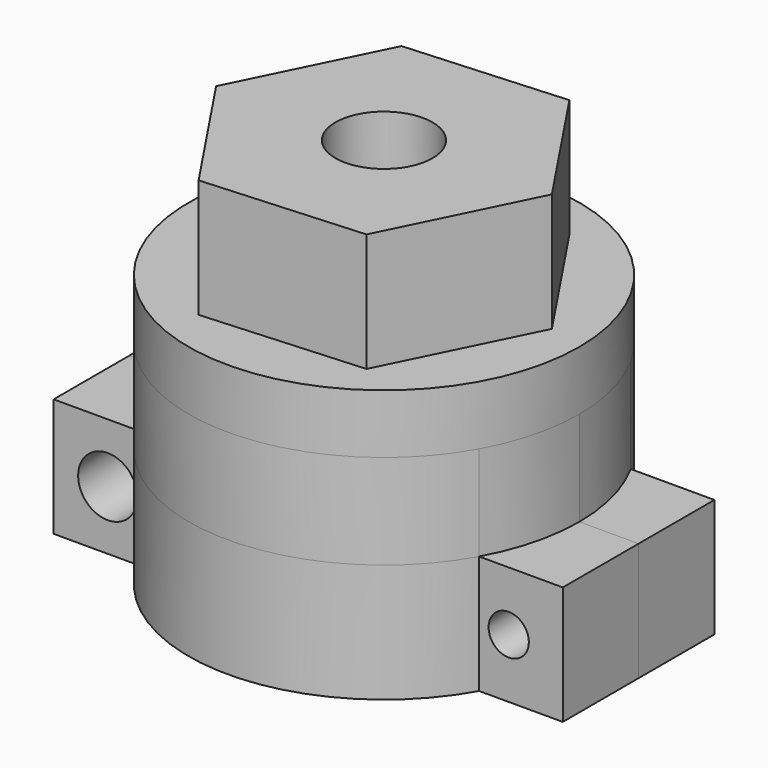
from build123d import *

# Parameters (mm, degrees)
F1_DEPTH       = 10
F2_DEPTH       = 10
F3_DEPTH       = 8
F5_D           = 3.4
F5_2_D         = 3.4
F7_D           = 5
F7_DEPTH       = 5
F7_TIP         = 1.5021515476
F7_ON_F6_D     = 5
F7_ON_F6_DEPTH = 5
F7_ON_F6_TIP   = 1.5021515476
F8_R           = 16.5
F8_R_2         = 10.5
F9_DEPTH       = 5
F11_DEPTH      = 10
F12_R          = 4.1
F13_DEPTH      = 13


# Not quite as in the source:
# - a feature names something its author has since deleted; it is built from what else it names


with BuildPart() as f1:
    # F0 (on Top) → F1 (new body)
    with BuildSketch(Plane.XY):
        with BuildLine():
            ThreePointArc((7.4833333333, 0.499722145), (7.4958321753, 0.25), (7.5, 0))
            Line((7.5, 0), (10.5, 0))
            ThreePointArc((10.5, 0), (0, 10.5), (-10.5, 0))
            Line((-10.5, 0), (-7.5, 0))
            ThreePointArc((-7.5, 0), (-7.4958321753, 0.25), (-7.4833333333, 0.499722145))
            ThreePointArc((-7.4833333333, 0.499722145), (-7.355889603, 1.4631774151), (-7.1049338873, 2.4020646238))
            ThreePointArc((-7.1049338873, 2.4020646238), (-7.020916784, 2.6375609021), (-6.9290964938, 2.8701257427))
            ThreePointArc((-6.9290964938, 2.8701257427), (-6.8295750678, 3.0995006684), (-6.7224631159, 3.3254307473))
            ThreePointArc((-6.7224631159, 3.3254307473), (-6.2360220923, 4.1667767476), (-5.6448726633, 4.9381588284))
            ThreePointArc((-5.6448726633, 4.9381588284), (-5.4771304571, 5.1235770665), (-5.3033008589, 5.3033008589))
            ThreePointArc((-5.3033008589, 5.3033008589), (-5.1235770665, 5.4771304571), (-4.9381588284, 5.6448726633))
            ThreePointArc((-4.9381588284, 5.6448726633), (-4.1667767476, 6.2360220923), (-3.3254307473, 6.7224631159))
            ThreePointArc((-3.3254307473, 6.7224631159), (-3.0995006684, 6.8295750678), (-2.8701257427, 6.9290964938))
            ThreePointArc((-2.8701257427, 6.9290964938), (-2.6375609021, 7.020916784), (-2.4020646238, 7.1049338873))
            ThreePointArc((-2.4020646238, 7.1049338873), (-1.4631774151, 7.355889603), (-0.499722145, 7.4833333333))
            ThreePointArc((-0.499722145, 7.4833333333), (-0.25, 7.4958321753), (0, 7.5))
            ThreePointArc((0, 7.5), (0.25, 7.4958321753), (0.499722145, 7.4833333333))
            ThreePointArc((0.499722145, 7.4833333333), (1.4631774151, 7.355889603), (2.4020646238, 7.1049338873))
            ThreePointArc((2.4020646238, 7.1049338873), (2.6375609021, 7.020916784), (2.8701257427, 6.9290964938))
            ThreePointArc((2.8701257427, 6.9290964938), (3.0995006684, 6.8295750678), (3.3254307473, 6.7224631159))
            ThreePointArc((3.3254307473, 6.7224631159), (4.1667767476, 6.2360220923), (4.9381588284, 5.6448726633))
            ThreePointArc((4.9381588284, 5.6448726633), (5.1235770665, 5.4771304571), (5.3033008589, 5.3033008589))
            ThreePointArc((5.3033008589, 5.3033008589), (5.4771304571, 5.1235770665), (5.6448726633, 4.9381588284))
            ThreePointArc((5.6448726633, 4.9381588284), (6.2360220923, 4.1667767476), (6.7224631159, 3.3254307473))
            ThreePointArc((6.7224631159, 3.3254307473), (6.8295750678, 3.0995006684), (6.9290964938, 2.8701257427))
            ThreePointArc((6.9290964938, 2.8701257427), (7.020916784, 2.6375609021), (7.1049338873, 2.4020646238))
            ThreePointArc((7.1049338873, 2.4020646238), (7.355889603, 1.4631774151), (7.4833333333, 0.499722145))
        make_face()
        with BuildLine():
            ThreePointArc((-10.5, 0), (0, 10.5), (10.5, 0))
            Line((10.5, 0), (16.5, 0))
            ThreePointArc((16.5, 0), (15.9743442726, 4.1316249903), (14.4308696897, 8))
            ThreePointArc((14.4308696897, 8), (0, 16.5), (-14.4308696897, 8))
            ThreePointArc((-14.4308696897, 8), (-15.9743442726, 4.1316249903), (-16.5, 0))
            Line((-16.5, 0), (-10.5, 0))
        make_face()
        with BuildLine():
            ThreePointArc((14.4308696897, 8), (15.9743442726, 4.1316249903), (16.5, 0))
            Line((16.5, 0), (21.5, 0))
            Line((21.5, 0), (21.5, 8))
            Line((21.5, 8), (14.4308696897, 8))
        make_face()
        with BuildLine():
            Line((-21.5, 0), (-16.5, 0))
            ThreePointArc((-16.5, 0), (-15.9743442726, 4.1316249903), (-14.4308696897, 8))
            Line((-14.4308696897, 8), (-21.5, 8))
            Line((-21.5, 8), (-21.5, 0))
        make_face()
        with BuildLine():
            ThreePointArc((-7.1049338873, 2.4020646238), (-7.355889603, 1.4631774151), (-7.4833333333, 0.499722145))
            Line((-7.4833333333, 0.499722145), (-6.3751043226, 1.2680870931))
            Line((-6.3751043226, 1.2680870931), (-7.1049338873, 2.4020646238))
        make_face()
        with BuildLine():
            ThreePointArc((-5.6448726633, 4.9381588284), (-6.2360220923, 4.1667767476), (-6.7224631159, 3.3254307473))
            Line((-6.7224631159, 3.3254307473), (-5.40455248, 3.6112065146))
            Line((-5.40455248, 3.6112065146), (-5.6448726633, 4.9381588284))
        make_face()
        with BuildLine():
            ThreePointArc((-3.3254307473, 6.7224631159), (-4.1667767476, 6.2360220923), (-4.9381588284, 5.6448726633))
            Line((-4.9381588284, 5.6448726633), (-3.6112065146, 5.40455248))
            Line((-3.6112065146, 5.40455248), (-3.3254307473, 6.7224631159))
        make_face()
        with BuildLine():
            Line((-1.2680870931, 6.3751043226), (-0.499722145, 7.4833333333))
            ThreePointArc((-0.499722145, 7.4833333333), (-1.4631774151, 7.355889603), (-2.4020646238, 7.1049338873))
            Line((-2.4020646238, 7.1049338873), (-1.2680870931, 6.3751043226))
        make_face()
        with BuildLine():
            Line((1.2680870931, 6.3751043226), (2.4020646238, 7.1049338873))
            ThreePointArc((2.4020646238, 7.1049338873), (1.4631774151, 7.355889603), (0.499722145, 7.4833333333))
            Line((0.499722145, 7.4833333333), (1.2680870931, 6.3751043226))
        make_face()
        with BuildLine():
            Line((3.6112065146, 5.40455248), (4.9381588284, 5.6448726633))
            ThreePointArc((4.9381588284, 5.6448726633), (4.1667767476, 6.2360220923), (3.3254307473, 6.7224631159))
            Line((3.3254307473, 6.7224631159), (3.6112065146, 5.40455248))
        make_face()
        with BuildLine():
            Line((5.40455248, 3.6112065146), (6.7224631159, 3.3254307473))
            ThreePointArc((6.7224631159, 3.3254307473), (6.2360220923, 4.1667767476), (5.6448726633, 4.9381588284))
            Line((5.6448726633, 4.9381588284), (5.40455248, 3.6112065146))
        make_face()
        with BuildLine():
            Line((6.3751043226, 1.2680870931), (7.4833333333, 0.499722145))
            ThreePointArc((7.4833333333, 0.499722145), (7.355889603, 1.4631774151), (7.1049338873, 2.4020646238))
            Line((7.1049338873, 2.4020646238), (6.3751043226, 1.2680870931))
        make_face()
    extrude(amount=-F1_DEPTH)

    # F0 (on Top) → F3 (join)
    with BuildSketch(Plane.XY):
        with BuildLine():
            Line((16.5, 0), (10.5, 0))
            ThreePointArc((10.5, 0), (0, -10.5), (-10.5, 0))
            Line((-10.5, 0), (-16.5, 0))
            ThreePointArc((-16.5, 0), (-15.9743442726, -4.1316249903), (-14.4308696897, -8))
            ThreePointArc((-14.4308696897, -8), (0, -16.5), (14.4308696897, -8))
            ThreePointArc((14.4308696897, -8), (15.9743442726, -4.1316249903), (16.5, 0))
        make_face()
        with BuildLine():
            ThreePointArc((-10.5, 0), (0, 10.5), (10.5, 0))
            Line((10.5, 0), (16.5, 0))
            ThreePointArc((16.5, 0), (15.9743442726, 4.1316249903), (14.4308696897, 8))
            ThreePointArc((14.4308696897, 8), (0, 16.5), (-14.4308696897, 8))
            ThreePointArc((-14.4308696897, 8), (-15.9743442726, 4.1316249903), (-16.5, 0))
            Line((-16.5, 0), (-10.5, 0))
        make_face()
    extrude(amount=F3_DEPTH)

    # F5 (through all)
    with Locations(Plane(origin=(0, 8, 0), x_dir=(-1, 0, 0), z_dir=(0, 1, 0))):
        with Locations((-16.9308696897, -5), (16.9308696897, -5)):
            Hole(F5_D / 2)

    # F7
    with Locations(Plane(origin=(0, 8, 0), x_dir=(-1, 0, 0), z_dir=(0, 1, 0))):
        with Locations((-16.9308696897, -5)):
            Hole(F7_D / 2, depth=F7_DEPTH)
            with Locations((0, 0, -(F7_DEPTH + F7_TIP / 2))):  # 118° drill point
                Cone(0, F7_D / 2, F7_TIP, mode=Mode.SUBTRACT)

    # F8 (on face) → F9 (join)
    with BuildSketch(Plane.XY.offset(8)):
        Circle(F8_R)
        Circle(F8_R_2, mode=Mode.SUBTRACT)
        Circle(F8_R_2)
    extrude(amount=F9_DEPTH)

    # F10 (on face) → F11 (join)
    with BuildSketch(Plane.XY.offset(13)):
        Polygon((-7.5000816839, 11.2249175826), (-13.4711046238, -0.8828024774), (-5.9710229399, -12.10772006), (7.5000816839, -11.2249175826), (13.4711046238, 0.8828024774), (5.9710229399, 12.10772006), align=None)
    extrude(amount=F11_DEPTH)

    # F12 (on face) → F13 (cut, through all)
    with BuildSketch(Plane.XY.offset(23)):
        Circle(F12_R)
    extrude(amount=-F13_DEPTH, mode=Mode.SUBTRACT)


with BuildPart() as f2:
    # F0 (on Top) → F2 (new body, through all)
    with BuildSketch(Plane.XY):
        with BuildLine():
            Line((10.5, 0), (7.5, 0))
            ThreePointArc((7.5, 0), (7.4958321753, -0.25), (7.4833333333, -0.499722145))
            ThreePointArc((7.4833333333, -0.499722145), (7.355889603, -1.4631774151), (7.1049338873, -2.4020646238))
            ThreePointArc((7.1049338873, -2.4020646238), (7.020916784, -2.6375609021), (6.9290964938, -2.8701257427))
            ThreePointArc((6.9290964938, -2.8701257427), (6.8295750678, -3.0995006684), (6.7224631159, -3.3254307473))
            ThreePointArc((6.7224631159, -3.3254307473), (6.2360220923, -4.1667767476), (5.6448726633, -4.9381588284))
            ThreePointArc((5.6448726633, -4.9381588284), (5.4771304571, -5.1235770665), (5.3033008589, -5.3033008589))
            ThreePointArc((5.3033008589, -5.3033008589), (5.1235770665, -5.4771304571), (4.9381588284, -5.6448726633))
            ThreePointArc((4.9381588284, -5.6448726633), (4.1667767476, -6.2360220923), (3.3254307473, -6.7224631159))
            ThreePointArc((3.3254307473, -6.7224631159), (3.0995006684, -6.8295750678), (2.8701257427, -6.9290964938))
            ThreePointArc((2.8701257427, -6.9290964938), (2.6375609021, -7.020916784), (2.4020646238, -7.1049338873))
            ThreePointArc((2.4020646238, -7.1049338873), (1.4631774151, -7.355889603), (0.499722145, -7.4833333333))
            ThreePointArc((0.499722145, -7.4833333333), (0.25, -7.4958321753), (0, -7.5))
            ThreePointArc((0, -7.5), (-0.25, -7.4958321753), (-0.499722145, -7.4833333333))
            ThreePointArc((-0.499722145, -7.4833333333), (-1.4631774151, -7.355889603), (-2.4020646238, -7.1049338873))
            ThreePointArc((-2.4020646238, -7.1049338873), (-2.6375609021, -7.020916784), (-2.8701257427, -6.9290964938))
            ThreePointArc((-2.8701257427, -6.9290964938), (-3.0995006684, -6.8295750678), (-3.3254307473, -6.7224631159))
            ThreePointArc((-3.3254307473, -6.7224631159), (-4.1667767476, -6.2360220923), (-4.9381588284, -5.6448726633))
            ThreePointArc((-4.9381588284, -5.6448726633), (-5.1235770665, -5.4771304571), (-5.3033008589, -5.3033008589))
            ThreePointArc((-5.3033008589, -5.3033008589), (-5.4771304571, -5.1235770665), (-5.6448726633, -4.9381588284))
            ThreePointArc((-5.6448726633, -4.9381588284), (-6.2360220923, -4.1667767476), (-6.7224631159, -3.3254307473))
            ThreePointArc((-6.7224631159, -3.3254307473), (-6.8295750678, -3.0995006684), (-6.9290964938, -2.8701257427))
            ThreePointArc((-6.9290964938, -2.8701257427), (-7.020916784, -2.6375609021), (-7.1049338873, -2.4020646238))
            ThreePointArc((-7.1049338873, -2.4020646238), (-7.355889603, -1.4631774151), (-7.4833333333, -0.499722145))
            ThreePointArc((-7.4833333333, -0.499722145), (-7.4958321753, -0.25), (-7.5, 0))
            Line((-7.5, 0), (-10.5, 0))
            ThreePointArc((-10.5, 0), (0, -10.5), (10.5, 0))
        make_face()
        with BuildLine():
            Line((16.5, 0), (10.5, 0))
            ThreePointArc((10.5, 0), (0, -10.5), (-10.5, 0))
            Line((-10.5, 0), (-16.5, 0))
            ThreePointArc((-16.5, 0), (-15.9743442726, -4.1316249903), (-14.4308696897, -8))
            ThreePointArc((-14.4308696897, -8), (0, -16.5), (14.4308696897, -8))
            ThreePointArc((14.4308696897, -8), (15.9743442726, -4.1316249903), (16.5, 0))
        make_face()
        with BuildLine():
            ThreePointArc((-14.4308696897, -8), (-15.9743442726, -4.1316249903), (-16.5, 0))
            Line((-16.5, 0), (-21.5, 0))
            Line((-21.5, 0), (-21.5, -8))
            Line((-21.5, -8), (-14.4308696897, -8))
        make_face()
        with BuildLine():
            Line((21.5, 0), (16.5, 0))
            ThreePointArc((16.5, 0), (15.9743442726, -4.1316249903), (14.4308696897, -8))
            Line((14.4308696897, -8), (21.5, -8))
            Line((21.5, -8), (21.5, 0))
        make_face()
        with BuildLine():
            Line((-6.3751043226, -1.2680870931), (-7.4833333333, -0.499722145))
            ThreePointArc((-7.4833333333, -0.499722145), (-7.355889603, -1.4631774151), (-7.1049338873, -2.4020646238))
            Line((-7.1049338873, -2.4020646238), (-6.3751043226, -1.2680870931))
        make_face()
        with BuildLine():
            Line((-5.40455248, -3.6112065146), (-6.7224631159, -3.3254307473))
            ThreePointArc((-6.7224631159, -3.3254307473), (-6.2360220923, -4.1667767476), (-5.6448726633, -4.9381588284))
            Line((-5.6448726633, -4.9381588284), (-5.40455248, -3.6112065146))
        make_face()
        with BuildLine():
            Line((-3.6112065146, -5.40455248), (-4.9381588284, -5.6448726633))
            ThreePointArc((-4.9381588284, -5.6448726633), (-4.1667767476, -6.2360220923), (-3.3254307473, -6.7224631159))
            Line((-3.3254307473, -6.7224631159), (-3.6112065146, -5.40455248))
        make_face()
        with BuildLine():
            Line((-1.2680870931, -6.3751043226), (-2.4020646238, -7.1049338873))
            ThreePointArc((-2.4020646238, -7.1049338873), (-1.4631774151, -7.355889603), (-0.499722145, -7.4833333333))
            Line((-0.499722145, -7.4833333333), (-1.2680870931, -6.3751043226))
        make_face()
        with BuildLine():
            ThreePointArc((0.499722145, -7.4833333333), (1.4631774151, -7.355889603), (2.4020646238, -7.1049338873))
            Line((2.4020646238, -7.1049338873), (1.2680870931, -6.3751043226))
            Line((1.2680870931, -6.3751043226), (0.499722145, -7.4833333333))
        make_face()
        with BuildLine():
            ThreePointArc((3.3254307473, -6.7224631159), (4.1667767476, -6.2360220923), (4.9381588284, -5.6448726633))
            Line((4.9381588284, -5.6448726633), (3.6112065146, -5.40455248))
            Line((3.6112065146, -5.40455248), (3.3254307473, -6.7224631159))
        make_face()
        with BuildLine():
            ThreePointArc((5.6448726633, -4.9381588284), (6.2360220923, -4.1667767476), (6.7224631159, -3.3254307473))
            Line((6.7224631159, -3.3254307473), (5.40455248, -3.6112065146))
            Line((5.40455248, -3.6112065146), (5.6448726633, -4.9381588284))
        make_face()
        with BuildLine():
            ThreePointArc((7.1049338873, -2.4020646238), (7.355889603, -1.4631774151), (7.4833333333, -0.499722145))
            Line((7.4833333333, -0.499722145), (6.3751043226, -1.2680870931))
            Line((6.3751043226, -1.2680870931), (7.1049338873, -2.4020646238))
        make_face()
    extrude(amount=-F2_DEPTH)

    # F5#2 (through all)
    with Locations(Plane(origin=(0, 8, 0), x_dir=(-1, 0, 0), z_dir=(0, 1, 0))):
        with Locations((-16.9308696897, -5), (16.9308696897, -5)):
            Hole(F5_2_D / 2)

    # F7 on F6
    with Locations(Plane.XZ.offset(8)):
        with Locations((-16.9308696897, -5)):
            Hole(F7_ON_F6_D / 2, depth=F7_ON_F6_DEPTH)
            with Locations((0, 0, -(F7_ON_F6_DEPTH + F7_ON_F6_TIP / 2))):  # 118° drill point
                Cone(0, F7_ON_F6_D / 2, F7_ON_F6_TIP, mode=Mode.SUBTRACT)


solid = Compound([f1.part, f2.part])
